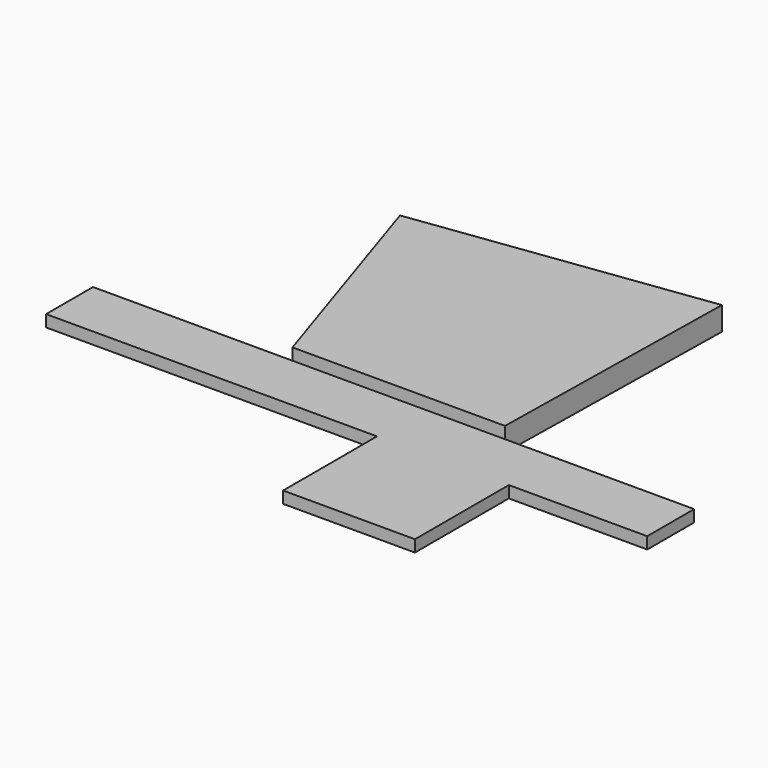
from build123d import *

# Parameters (mm, degrees)
F1_DEPTH = 1
F2_W     = 5.6130217854
F2_H     = 2.4976935238
F2_W_2   = 14.08868609
F2_W_3   = 5.8936730493
F2_H_2   = 4.9955896102
F3_DEPTH = 0.5


with BuildPart() as f1:
    # F0 (on Top) → F1 (new body)
    with BuildSketch(Plane.XY):
        Polygon((-12.1924033149, 9.6513108647), (-9.05, 0), (-5.4919267763, 4.3473211306), align=None)
        Polygon((-5.4919267763, 4.3473211306), (0, 0), (0.1970994475, 11.2982809227), align=None)
        Polygon((-12.1924033149, 9.6513108647), (-5.4919267763, 4.3473211306), (0.1970994475, 11.2982809227), align=None)
        Polygon((-9.05, 0), (0, 0), (-5.4919267763, 4.3473211306), align=None)
    extrude(amount=F1_DEPTH)

    # F2 (on Top) → F3 (join)
    with BuildSketch(Plane.XY):
        with Locations((-0.6455987459, -1.2488467619)):
            Rectangle(F2_W, F2_H)
        with Locations((-10.4964526836, -1.2488467619)):
            Rectangle(F2_W_2, F2_H)
        with Locations((5.1077486714, -1.2488467619)):
            Rectangle(F2_W_3, F2_H)
        with Locations((-0.6455987459, -4.9954883289)):
            Rectangle(F2_W, F2_H_2)
    extrude(amount=F3_DEPTH)


solid = f1.part
